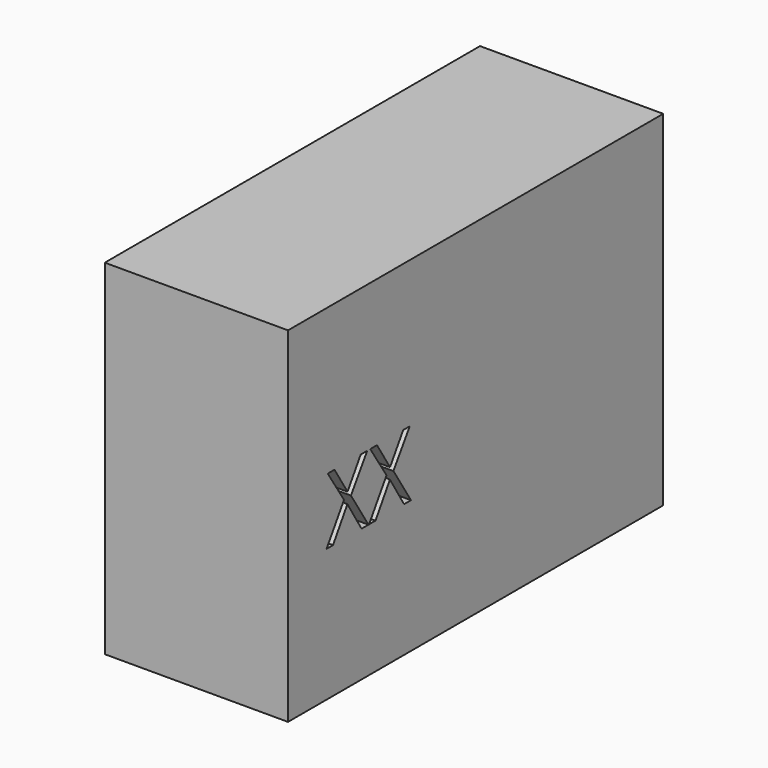
from build123d import *

# Parameters (mm, degrees)
F0_W         = 63.9843791723
F0_H         = 47.031249851
F1_DEPTH     = 25
F2_TEXT_SIZE = 12.5572137121
F3_DEPTH     = 3


# Not quite as in the source:
# - a feature of the source that left no trace in its solid (it failed there, or was rolled back) is left out
# - Text() gives the source's letters only with a copy of the font that has no kerning and outlines rounded to 1/6400 em; it was checked with that copy


with BuildPart() as f1:
    # F0 (on Right) → F1 (new body)
    with BuildSketch(Plane.YZ):
        with Locations((-31.9921895862, 23.5156249255)):
            Rectangle(F0_W, F0_H)
    extrude(amount=F1_DEPTH)

    # F2 (on face) → F3 (cut)
    with BuildSketch(Plane.YZ.offset(25)):
        with Locations((-57.464953512, 18.1078780442)):
            Text('XX', F2_TEXT_SIZE, font='Open Sans', text_align=(TextAlign.LEFT, TextAlign.BOTTOM))
    extrude(amount=-F3_DEPTH, mode=Mode.SUBTRACT)


solid = f1.part
